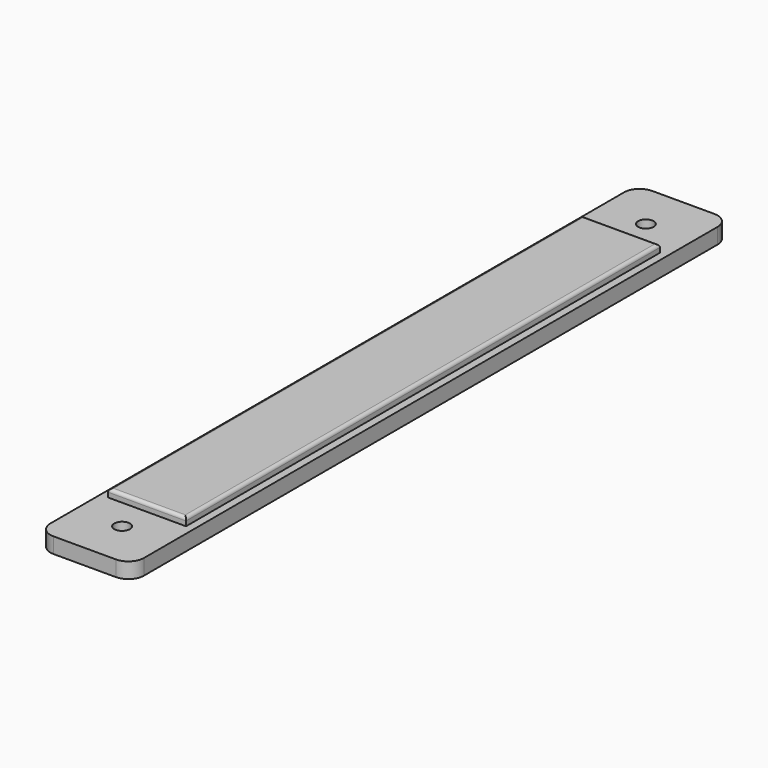
from build123d import *

# Parameters (mm, degrees)
F1_DEPTH = 3.175
F2_D     = 3.175
F3_W     = 15.875
F3_H     = 120.65
F4_DEPTH = 1.5875
F5_R     = 0.635


# Not quite as in the source:
# - a feature names something its author has since deleted; it is built from what else it names


with BuildPart() as f1:
    # F0 (on Top) → F1 (new body)
    with BuildSketch(Plane.XY):
        with BuildLine():
            Line((6.35, 76.2), (-6.35, 76.2))
            ThreePointArc((-6.35, 76.2), (-8.5950640303, 75.2700640303), (-9.525, 73.025))
            Line((-9.525, 73.025), (-9.525, -73.025))
            ThreePointArc((-9.525, -73.025), (-8.5950640303, -75.2700640303), (-6.35, -76.2))
            Line((-6.35, -76.2), (6.35, -76.2))
            ThreePointArc((6.35, -76.2), (8.5950640303, -75.2700640303), (9.525, -73.025))
            Line((9.525, -73.025), (9.525, 73.025))
            ThreePointArc((9.525, 73.025), (8.5950640303, 75.2700640303), (6.35, 76.2))
        make_face()
    extrude(amount=F1_DEPTH)

    # F2 (through all)
    with Locations(Plane(origin=(0, 0, 0), x_dir=(1, 0, 0), z_dir=(0, 0, -1))):
        with Locations((0, 66.675), (0, -66.675)):
            Hole(F2_D / 2)

    # F3 (on face) → F4 (join)
    with BuildSketch(Plane.XY.offset(3.175)):
        Rectangle(F3_W, F3_H)
    extrude(amount=F4_DEPTH)

    # F5
    f5_edges = [f1.edges().sort_by_distance(p)[0] for p in [
        (0, -60.325, 4.7625),
        (7.9375, 0, 4.7625),
        (-7.9375, 0, 4.7625),
        (0, 60.325, 4.7625),
    ]]
    fillet(f5_edges, radius=F5_R)


solid = f1.part
